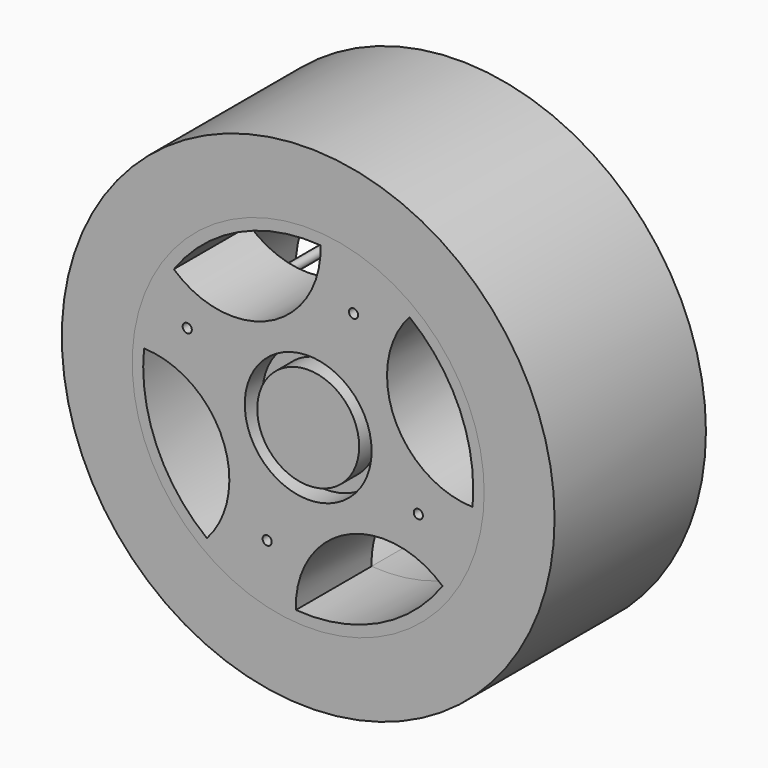
from build123d import *
from build123d import SkipClean  # not in build123d's __all__

# Parameters (mm, degrees)
F0_R      = 24
F0_R_2    = 0.6247236377
F0_R_3    = 8.65
F1_DEPTH  = 12.9
F2_DEPTH  = 12.9
F0_R_4    = 6.95
F0_W      = 5.5
F0_H      = 3.7
F3_DEPTH  = 12.9
F4_DEPTH  = 9.9
F5_DEPTH  = 9.9
F6_DEPTH  = 18.3
F7_DEPTH  = 5
F8_R      = 33.6
F8_R_2    = 24
F9_DEPTH  = 12.9
F10_DEPTH = 12.9
F11_DEPTH = 11


# Not quite as in the source:
# - a feature names something its author has since deleted; it is built from what else it names


with BuildPart() as f1:
    # F0 (on Front) → F1 (new body)
    with BuildSketch(Plane.XZ):
        Circle(F0_R)
        with BuildLine():
            ThreePointArc((13.8107888925, 17.76266056), (20.211293255, 9.887043287), (22.5, 0))
            ThreePointArc((22.5, 0), (22.4721042456, -1.1200583811), (22.3884861532, -2.23733944))
            ThreePointArc((22.3884861532, -2.23733944), (21.0615108713, -7.9159812923), (18.3197080891, -13.0628593934))
            ThreePointArc((18.3197080891, -13.0628593934), (9.5491868643, -20.3730957449), (-1.6802919109, -22.4371704788))
            ThreePointArc((-1.6802919109, -22.4371704788), (-8.0904979364, -20.9950909296), (-13.8107888925, -17.76266056))
            ThreePointArc((-13.8107888925, -17.76266056), (-20.6784157627, -8.8686595122), (-22.3884861532, 2.23733944))
            ThreePointArc((-22.3884861532, 2.23733944), (-21.0615108713, 7.9159812923), (-18.3197080891, 13.0628593934))
            ThreePointArc((-18.3197080891, 13.0628593934), (-9.5491868643, 20.3730957449), (1.6802919109, 22.4371704788))
            ThreePointArc((1.6802919109, 22.4371704788), (8.0904979364, 20.9950909296), (13.8107888925, 17.76266056))
        make_face(mode=Mode.SUBTRACT)
        with BuildLine():
            ThreePointArc((22.3884861532, -2.23733944), (11.7216927981, 5.0272566102), (13.8107888925, 17.76266056))
            ThreePointArc((13.8107888925, 17.76266056), (8.0904979364, 20.9950909296), (1.6802919109, 22.4371704788))
            ThreePointArc((1.6802919109, 22.4371704788), (-5.218842533, 11.134348936), (-18.3197080891, 13.0628593934))
            ThreePointArc((-18.3197080891, 13.0628593934), (-21.0615108713, 7.9159812923), (-22.3884861532, 2.23733944))
            ThreePointArc((-22.3884861532, 2.23733944), (-11.7216927981, -5.0272566102), (-13.8107888925, -17.76266056))
            ThreePointArc((-13.8107888925, -17.76266056), (-8.0904979364, -20.9950909296), (-1.6802919109, -22.4371704788))
            ThreePointArc((-1.6802919109, -22.4371704788), (5.218842533, -11.134348936), (18.3197080891, -13.0628593934))
            ThreePointArc((18.3197080891, -13.0628593934), (21.0615108713, -7.9159812923), (22.3884861532, -2.23733944))
        make_face()
        with Locations((-5.5955685675, -15.3557388112)):
            Circle(F0_R_2, mode=Mode.SUBTRACT)
        with Locations((15.0192249566, -5.4900874384)):
            Circle(F0_R_2, mode=Mode.SUBTRACT)
        with Locations((-16.4919588715, 6.584291812)):
            Circle(F0_R_2, mode=Mode.SUBTRACT)
        Circle(F0_R_3, mode=Mode.SUBTRACT)
        with Locations((6.1843143776, 15.7137010247)):
            Circle(F0_R_2, mode=Mode.SUBTRACT)
    extrude(amount=F1_DEPTH)

    # F0 (on Front) → F2 (join)
    with BuildSketch(Plane.XZ):
        Circle(F0_R)
        with BuildLine():
            ThreePointArc((13.8107888925, 17.76266056), (20.211293255, 9.887043287), (22.5, 0))
            ThreePointArc((22.5, 0), (22.4721042456, -1.1200583811), (22.3884861532, -2.23733944))
            ThreePointArc((22.3884861532, -2.23733944), (21.0615108713, -7.9159812923), (18.3197080891, -13.0628593934))
            ThreePointArc((18.3197080891, -13.0628593934), (9.5491868643, -20.3730957449), (-1.6802919109, -22.4371704788))
            ThreePointArc((-1.6802919109, -22.4371704788), (-8.0904979364, -20.9950909296), (-13.8107888925, -17.76266056))
            ThreePointArc((-13.8107888925, -17.76266056), (-20.6784157627, -8.8686595122), (-22.3884861532, 2.23733944))
            ThreePointArc((-22.3884861532, 2.23733944), (-21.0615108713, 7.9159812923), (-18.3197080891, 13.0628593934))
            ThreePointArc((-18.3197080891, 13.0628593934), (-9.5491868643, 20.3730957449), (1.6802919109, 22.4371704788))
            ThreePointArc((1.6802919109, 22.4371704788), (8.0904979364, 20.9950909296), (13.8107888925, 17.76266056))
        make_face(mode=Mode.SUBTRACT)
    with SkipClean():  # cleaning this boolean's faces spoils the solid; the shape is the same uncleaned
        extrude(amount=-F2_DEPTH)


with BuildPart() as f3:
    # F0 (on Front) → F3 (new body)
    with BuildSketch(Plane.XZ):
        Circle(F0_R_4)
        Rectangle(F0_W, F0_H, mode=Mode.SUBTRACT)
        Rectangle(F0_W, F0_H)
    extrude(amount=F3_DEPTH)

    # F0 (on Front) → F7 (join)
    with BuildSketch(Plane.XZ):
        Rectangle(F0_W, F0_H)
    extrude(amount=-F7_DEPTH)


with BuildPart() as f4:
    # F0 (on Front) → F4 (new body)
    with BuildSketch(Plane.XZ):
        Circle(F0_R_3)
        Circle(F0_R_4, mode=Mode.SUBTRACT)
    extrude(amount=F4_DEPTH)


with BuildPart() as f5:
    # F0 (on Front) → F5 (new body)
    with BuildSketch(Plane.XZ):
        Circle(F0_R_3)
        Circle(F0_R_4, mode=Mode.SUBTRACT)
    extrude(amount=F5_DEPTH)


with BuildPart() as f6:
    # F0 (on Front) → F6 (new body)
    with BuildSketch(Plane.XZ):
        Circle(F0_R_4)
        Rectangle(F0_W, F0_H, mode=Mode.SUBTRACT)
    extrude(amount=-F6_DEPTH)


with BuildPart() as f9:
    # F8 (on Front) → F9 (new body)
    with BuildSketch(Plane.XZ):
        Circle(F8_R)
        Circle(F8_R_2, mode=Mode.SUBTRACT)
    extrude(amount=F9_DEPTH)

    # F10 (add): a face of the model
    f10_faces = [f9.faces().sort_by_distance(p)[0] for p in [
        (-32.6496484861, 0, 0),
    ]]
    extrude(f10_faces, amount=F10_DEPTH)


with BuildPart() as f11:
    # F0 (on Front) → F11 (new body)
    with BuildSketch(Plane.XZ):
        with Locations((6.1843143776, 15.7137010247)):
            Circle(F0_R_2)
    extrude(amount=-F11_DEPTH)


with BuildPart() as f11b:
    # F0 (on Front) → F11, piece 2 (new body)
    with BuildSketch(Plane.XZ):
        with Locations((-16.4919588715, 6.584291812)):
            Circle(F0_R_2)
    extrude(amount=-F11_DEPTH)


with BuildPart() as f11c:
    # F0 (on Front) → F11, piece 3 (new body)
    with BuildSketch(Plane.XZ):
        with Locations((15.0192249566, -5.4900874384)):
            Circle(F0_R_2)
    extrude(amount=-F11_DEPTH)


with BuildPart() as f11d:
    # F0 (on Front) → F11, piece 4 (new body)
    with BuildSketch(Plane.XZ):
        with Locations((-5.5955685675, -15.3557388112)):
            Circle(F0_R_2)
    extrude(amount=-F11_DEPTH)


solid = Compound([f1.part, f3.part, f4.part, f5.part, f6.part, f9.part, f11.part, f11b.part, f11c.part, f11d.part])
